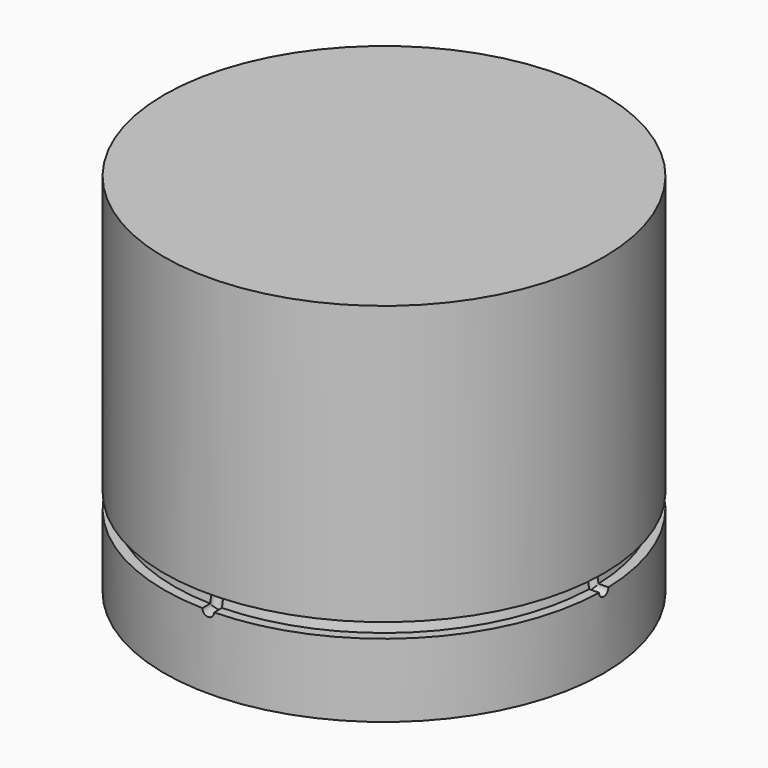
from build123d import *

# Parameters (mm, degrees)
F5_R     = 2
F7_COUNT = 4
F7_ANGLE = 270


# Not quite as in the source:
# - ends of sketch curves that miss each other by under 0.0002 mm in the source are joined


with BuildPart() as f1:
    # F0 (on Front) → F1 (revolve)
    with BuildSketch(Plane.XZ):
        with BuildLine():
            Line((-16.75, -14.0521210985), (0, -14.0521210985))
            Line((0, -14.0521210985), (0, -9.7755804438))
            Line((0, -9.7755804438), (0, 34.4478789015))
            Line((0, 34.4478789015), (-15.6576660306, 34.4478789015))
            ThreePointArc((-15.6576660306, 34.4478789015), (-18.0925700135, 33.4620870461), (-19.1558691306, 31.0600175269))
            Line((-19.1558691306, 31.0600175269), (-20.1051177665, 1.4478789015))
            Line((-20.1051177665, 1.4478789015), (-25.3049040659, -17.9579877563))
            ThreePointArc((-25.3049040659, -17.9579877563), (-26.5549794564, -19.8288577895), (-28.6856444579, -20.5521210985))
            Line((-28.6856444579, -20.5521210985), (-42, -20.5521210985))
            Line((-42, -20.5521210985), (-42, -30.5521210985))
            Line((-42, -30.5521210985), (-22.0613894912, -30.5521210985))
            Line((-22.0613894912, -30.5521210985), (-16.75, -22.0521210985))
            Line((-16.75, -22.0521210985), (-16.75, -14.0521210985))
        make_face()
        with BuildLine():
            Line((-47, -30.5521210985), (-42, -30.5521210985))
            Line((-42, -30.5521210985), (-42, -20.5521210985))
            Line((-42, -20.5521210985), (-54.0571891388, -25.9949319596))
            ThreePointArc((-54.0571891388, -25.9949319596), (-49.2876159651, -26.351767203), (-47, -30.5521210985))
        make_face()
        with BuildLine():
            Line((-57, -30.5521210985), (-47, -30.5521210985))
            ThreePointArc((-47, -30.5521210985), (-49.2876159651, -26.351767203), (-54.0571891388, -25.9949319596))
            ThreePointArc((-54.0571891388, -25.9949319596), (-56.2003538955, -27.8397370635), (-57, -30.5521210985))
        make_face()
        with BuildLine():
            ThreePointArc((-52, -35.5521210985), (-48.4644660941, -34.0876550044), (-47, -30.5521210985))
            Line((-47, -30.5521210985), (-57, -30.5521210985))
            ThreePointArc((-57, -30.5521210985), (-55.5355339059, -34.0876550044), (-52, -35.5521210985))
        make_face()
        with BuildLine():
            Line((-42, -35.5521210985), (-42, -30.5521210985))
            Line((-42, -30.5521210985), (-47, -30.5521210985))
            ThreePointArc((-47, -30.5521210985), (-48.4644660941, -34.0876550044), (-52, -35.5521210985))
            Line((-52, -35.5521210985), (-42, -35.5521210985))
        make_face()
        Polygon((-25.1857362508, -35.5521210985), (-22.0613894912, -30.5521210985), (-42, -30.5521210985), (-42, -35.5521210985), align=None)
    revolve(axis=Axis((0, 0, 11.9478789015), (0, 0, 1)))


with BuildPart() as f2:
    # F0 (on Front) → F2 (revolve)
    with BuildSketch(Plane.XZ):
        with BuildLine():
            Line((0, -70.5521210985), (0, -30.5521210985))
            Line((0, -30.5521210985), (-22.0613894912, -30.5521210985))
            Line((-22.0613894912, -30.5521210985), (-25.1857362508, -35.5521210985))
            Line((-25.1857362508, -35.5521210985), (-42, -35.5521210985))
            Line((-42, -35.5521210985), (-52, -35.5521210985))
            ThreePointArc((-52, -35.5521210985), (-55.5355339059, -34.0876550044), (-57, -30.5521210985))
            Line((-57, -30.5521210985), (-60, -30.5521210985))
            ThreePointArc((-60, -30.5521210985), (-62, -32.5521210985), (-64, -30.5521210985))
            Line((-64, -30.5521210985), (-69, -30.5521210985))
            Line((-69, -30.5521210985), (-70.7632698071, -40.5521210985))
            Line((-70.7632698071, -40.5521210985), (-71.6449047106, -45.5521210985))
            Line((-71.6449047106, -45.5521210985), (-75, -45.5521210985))
            Line((-75, -45.5521210985), (-75, -70.5521210985))
            Line((-75, -70.5521210985), (0, -70.5521210985))
        make_face()
        Polygon((0, -30.5521210985), (0, -14.0521210985), (-16.75, -14.0521210985), (-16.75, -22.0521210985), (-22.0613894912, -30.5521210985), align=None)
    revolve(axis=Axis((0, 0, 11.9478789015), (0, 0, 1)))

    # F6: sweep along a path in F0
    with BuildLine(Plane.XZ) as f6_path:
        Line((-75, -45.5521210985), (-71.6449047106, -45.5521210985))
        Line((-71.6449047106, -45.5521210985), (-69, -30.5521210985))
        Line((-69, -30.5521210985), (-62, -30.5521210985))
    # F5 (on offset) → F6 (sweep, cut)
    with BuildSketch(Plane.YZ.offset(-75)):
        with Locations((0, -45.5517880619)):
            Circle(F5_R)
    f6 = sweep(path=f6_path.line, transition=Transition.RIGHT, mode=Mode.SUBTRACT)

    # F7: F6 ×4 about axis
    f7_axis = Axis((0, 0, 11.9478789015), (0, 0, 1))
    for i in range(1, F7_COUNT):
        add(f6.rotate(f7_axis, i * F7_ANGLE / (F7_COUNT - 1)), mode=Mode.SUBTRACT)


with BuildPart() as f3:
    # F0 (on Front) → F3 (revolve)
    with BuildSketch(Plane.XZ):
        with BuildLine():
            Line((-15.6576660306, 34.4478789015), (0, 34.4478789015))
            Line((0, 34.4478789015), (0, 54.4478789015))
            Line((0, 54.4478789015), (-75, 54.4478789015))
            Line((-75, 54.4478789015), (-75, -30.5521210985))
            Line((-75, -30.5521210985), (-69, -30.5521210985))
            Line((-69, -30.5521210985), (-64, -30.5521210985))
            ThreePointArc((-64, -30.5521210985), (-62, -28.5521210985), (-60, -30.5521210985))
            Line((-60, -30.5521210985), (-57, -30.5521210985))
            ThreePointArc((-57, -30.5521210985), (-56.2003538955, -27.8397370635), (-54.0571891388, -25.9949319596))
            Line((-54.0571891388, -25.9949319596), (-42, -20.5521210985))
            Line((-42, -20.5521210985), (-28.6856444579, -20.5521210985))
            ThreePointArc((-28.6856444579, -20.5521210985), (-26.5549794564, -19.8288577895), (-25.3049040659, -17.9579877563))
            Line((-25.3049040659, -17.9579877563), (-20.1051177665, 1.4478789015))
            Line((-20.1051177665, 1.4478789015), (-19.1558691306, 31.0600175269))
            ThreePointArc((-19.1558691306, 31.0600175269), (-18.0925700135, 33.4620870461), (-15.6576660306, 34.4478789015))
        make_face()
        Polygon((-69, -30.5521210985), (-75, -30.5521210985), (-75, -40.5521210985), (-70.7632698071, -40.5521210985), align=None)
        with BuildLine():
            Line((-62, -30.5521210985), (-60, -30.5521210985))
            ThreePointArc((-60, -30.5521210985), (-62, -28.5521210985), (-64, -30.5521210985))
            Line((-64, -30.5521210985), (-62, -30.5521210985))
        make_face()
    revolve(axis=Axis((0, 0, 11.9478789015), (0, 0, 1)))


solid = Compound([f1.part, f2.part, f3.part])
